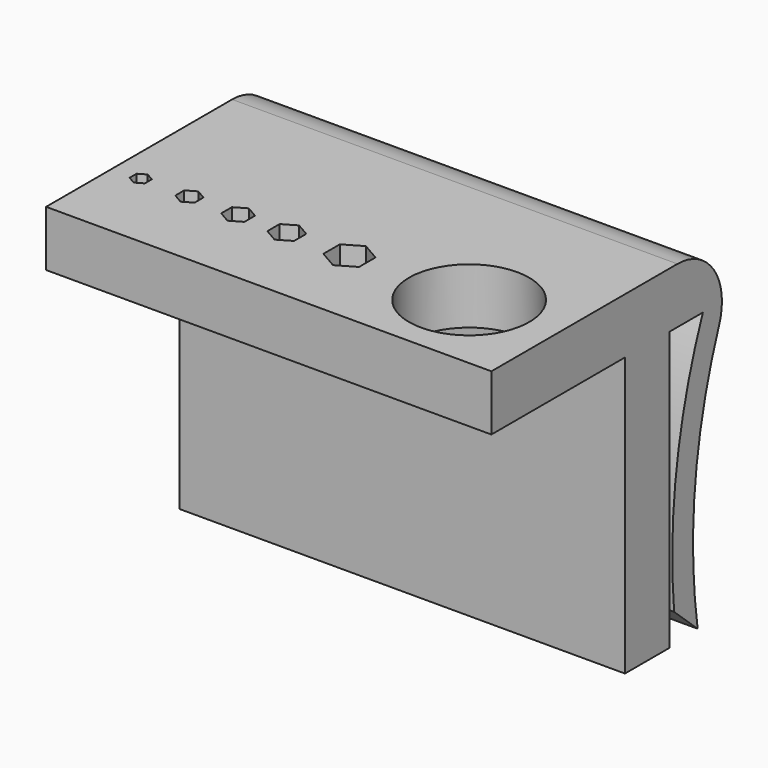
from build123d import *

# Parameters (mm, degrees)
F0_W        = 19.05
F0_H        = 6.35
F0_W_2      = 6.35
F0_H_2      = 31.75
F1_DEPTH    = 50.8
F3_DEPTH    = 38.101
F4_R        = 6.35
F5_T1_DEPTH = 68.1131376889


# Not quite as in the source:
# - a fillet or chamfer that OpenCascade refuses, or shapes differently, is made with other operations: its cross-section is extruded or revolved along the edge and cut away or added


with BuildPart() as f1:
    # F0 (on Right) → F1 (new body)
    with BuildSketch(Plane.YZ):
        with Locations((-15.875, 47.625)):
            Rectangle(F0_W, F0_H)
        with Locations((-3.175, 47.625)):
            Rectangle(F0_W_2, F0_H)
        with Locations((-3.175, 28.575)):
            Rectangle(F0_W_2, F0_H_2)
        with BuildLine():
            Line((0, 50.8), (0, 44.45))
            Line((0, 44.45), (4.7625, 44.45))
            ThreePointArc((4.7625, 44.45), (0.8082593776, 28.8201935432), (1.0656091525, 12.7))
            Line((1.0656091525, 12.7), (4.0578971116, 12.7))
            ThreePointArc((4.0578971116, 12.7), (4.3300087855, 32.3527315264), (11.1125, 50.8))
            Line((11.1125, 50.8), (0, 50.8))
        make_face()
    extrude(amount=F1_DEPTH)

    # F2 (on face) → F3 (cut, through all)
    with BuildSketch(Plane.XY.offset(50.8)):
        Polygon((2.3061167124, -15.875), (3.175, -15.875), (4.0438832876, -15.875), (4.0438832876, -15.37335), (3.175, -14.8717), (2.3061167124, -15.37335), align=None)
        Polygon((4.0438832876, -15.875), (3.175, -15.875), (2.3061167124, -15.875), (2.3061167124, -16.37665), (3.175, -16.8783), (4.0438832876, -16.37665), align=None)
        with BuildLine():
            ThreePointArc((47.498, -15.875), (40.64, -9.017), (33.782, -15.875))
            Line((33.782, -15.875), (40.64, -15.875))
            Line((40.64, -15.875), (47.498, -15.875))
        make_face()
        with BuildLine():
            Line((40.64, -15.875), (33.782, -15.875))
            ThreePointArc((33.782, -15.875), (40.64, -22.733), (47.498, -15.875))
            Line((47.498, -15.875), (40.64, -15.875))
        make_face()
        Polygon((24.9555, -14.701824253), (24.9555, -15.875), (26.9875, -15.875), (29.0195, -15.875), (29.0195, -14.701824253), (26.9875, -13.528648506), align=None)
        Polygon((26.9875, -15.875), (24.9555, -15.875), (24.9555, -17.048175747), (26.9875, -18.221351494), (29.0195, -17.048175747), (29.0195, -15.875), align=None)
        Polygon((18.3259538773, -14.9987), (18.3259538773, -15.875), (19.84375, -15.875), (21.3615461227, -15.875), (21.3615461227, -14.9987), (19.84375, -14.1224), align=None)
        Polygon((19.84375, -15.875), (18.3259538773, -15.875), (18.3259538773, -16.7513), (19.84375, -17.6276), (21.3615461227, -16.7513), (21.3615461227, -15.875), align=None)
        Polygon((12.9676772846, -15.113), (12.9676772846, -15.875), (14.2875, -15.875), (15.6073227154, -15.875), (15.6073227154, -15.113), (14.2875, -14.351), align=None)
        Polygon((14.2875, -15.875), (12.9676772846, -15.875), (12.9676772846, -16.637), (14.2875, -17.399), (15.6073227154, -16.637), (15.6073227154, -15.875), align=None)
        Polygon((7.6313977372, -15.24), (7.6313977372, -15.875), (8.73125, -15.875), (9.8311022628, -15.875), (9.8311022628, -15.24), (8.73125, -14.605), align=None)
        Polygon((8.73125, -15.875), (7.6313977372, -15.875), (7.6313977372, -16.51), (8.73125, -17.145), (9.8311022628, -16.51), (9.8311022628, -15.875), align=None)
    extrude(amount=-F3_DEPTH, mode=Mode.SUBTRACT)

    # F4
    f4_edges = [f1.edges().sort_by_distance(p)[0] for p in [
        (25.4, 11.1125, 50.8),
    ]]
    fillet(f4_edges, radius=F4_R)

    # F5: chamfer of 3.175 on 1 edges, made by hand

    # F5_s2 → F5_t1 (cut)
    with BuildSketch(Plane.YZ.offset(-8.6565688444)):
        with BuildLine():
            Line((4.422273237, 12.6144658264), (0.5675477916, 16.1266199594))
            Line((0.5675477916, 16.1266199594), (0.5043218231, 16.1207270056))
            ThreePointArc((0.5043218231, 16.1207270056), (0.7717830499, 14.4079265456), (1.0028018544, 12.690646214))
            Line((1.0028018544, 12.690646214), (1.0656091525, 12.6365))
            ThreePointArc((1.0656091525, 12.6365), (2.7439411948, 12.6365), (4.422273237, 12.5509658264))
            Line((4.422273237, 12.5509658264), (4.422273237, 12.6144658264))
        make_face()
    extrude(amount=F5_T1_DEPTH, mode=Mode.SUBTRACT)


solid = f1.part
